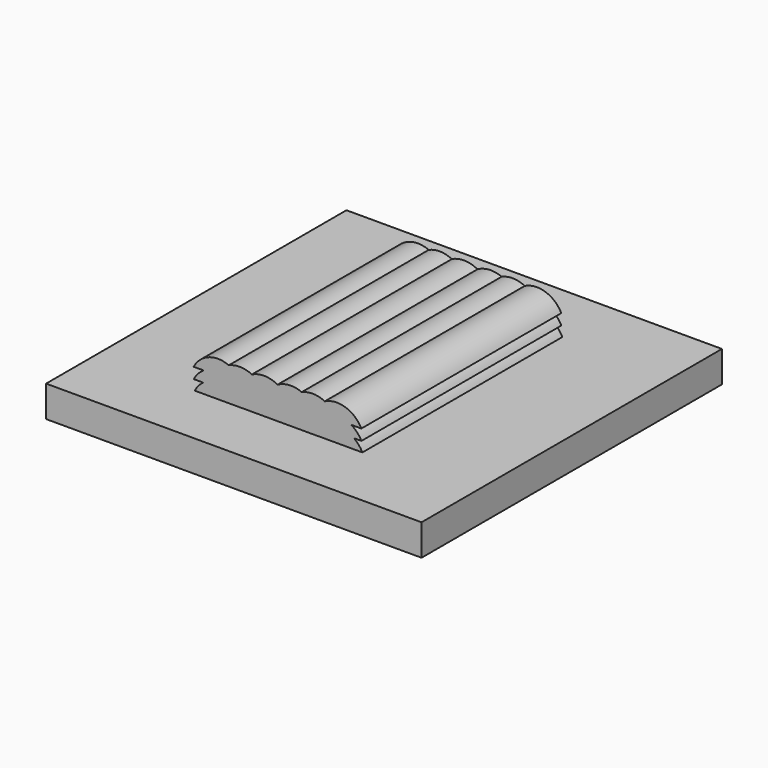
from build123d import *

# Parameters (mm, degrees)
F0_W     = 152.6275277138
F0_H     = 152.6275202632
F1_DEPTH = 12.7
F4_DEPTH = 101.6


with BuildPart() as f1:
    # F0 (on Top) → F1 (new body)
    with BuildSketch(Plane.XY):
        with Locations((0.3492608666, -0.1746304333)):
            Rectangle(F0_W, F0_H)
    extrude(amount=F1_DEPTH)


with BuildPart() as f4:
    # F3 (on offset) → F4 (new body)
    with BuildSketch(Plane.XZ.offset(50.8)):
        with BuildLine():
            ThreePointArc((-23.899851243, 16.6892502457), (-25.8361923758, 14.9089254969), (-27.3004854098, 12.7237895504))
            Line((-27.3004854098, 12.7237895504), (-17.3901738599, 12.7237895504))
            ThreePointArc((-17.3901738599, 12.7237895504), (-15.911695575, 14.925434135), (-13.9541862477, 16.7146502063))
            Line((-13.9541862477, 16.7146502063), (-16.6790850963, 16.7146502063))
            ThreePointArc((-16.6790850963, 16.7146502063), (-16.6725748067, 16.7019543949), (-16.6660808027, 16.6892502457))
            Line((-16.6660808027, 16.6892502457), (-19.7101641502, 16.6892502457))
            Line((-19.7101641502, 16.6892502457), (-23.899851243, 16.6892502457))
        make_face()
        with BuildLine():
            Line((-17.3901738599, 12.7237895504), (-27.3004854098, 12.7237895504))
            ThreePointArc((-27.3004854098, 12.7237895504), (-25.8361923758, 14.9089254969), (-23.899851243, 16.6892502457))
            Line((-23.899851243, 16.6892502457), (-32.6588120256, 16.6892502457))
            ThreePointArc((-32.6588120256, 16.6892502457), (-34.6163213529, 14.9000341745), (-36.0947996378, 12.6983895898))
            Line((-36.0947996378, 12.6983895898), (-16.274176538, 12.6983895898))
            ThreePointArc((-16.274176538, 12.6983895898), (-16.280670542, 12.711093739), (-16.2871808316, 12.7237895504))
            Line((-16.2871808316, 12.7237895504), (-17.3901738599, 12.7237895504))
        make_face()
        with BuildLine():
            ThreePointArc((-13.9541862477, 16.7146502063), (-15.911695575, 14.925434135), (-17.3901738599, 12.7237895504))
            Line((-17.3901738599, 12.7237895504), (-16.2871808316, 12.7237895504))
            Line((-16.2871808316, 12.7237895504), (-7.47986231, 12.7237895504))
            Line((-7.47986231, 12.7237895504), (-6.4638601616, 12.7237895504))
            ThreePointArc((-6.4638601616, 12.7237895504), (-4.9853818767, 14.925434135), (-3.0278725494, 16.7146502063))
            Line((-3.0278725494, 16.7146502063), (-6.8557644263, 16.7146502063))
            Line((-6.8557644263, 16.7146502063), (-7.8717665747, 16.7146502063))
            Line((-7.8717665747, 16.7146502063), (-13.9541862477, 16.7146502063))
        make_face()
        with BuildLine():
            ThreePointArc((-23.8644977976, 16.7146502063), (-23.8821869424, 16.701967516), (-23.899851243, 16.6892502457))
            Line((-23.899851243, 16.6892502457), (-19.7101641502, 16.6892502457))
            ThreePointArc((-19.7101641502, 16.6892502457), (-19.7279755385, 16.7019677558), (-19.7458119078, 16.7146502063))
            Line((-19.7458119078, 16.7146502063), (-23.8644977976, 16.7146502063))
        make_face()
        with BuildLine():
            Line((-32.6588120256, 16.6892502457), (-23.899851243, 16.6892502457))
            ThreePointArc((-23.899851243, 16.6892502457), (-23.8821869424, 16.701967516), (-23.8644977976, 16.7146502063))
            Line((-23.8644977976, 16.7146502063), (-27.6923896745, 16.7146502063))
            ThreePointArc((-27.6923896745, 16.7146502063), (-25.9698422833, 19.1904969058), (-23.6456289265, 21.1127400398))
            Line((-23.6456289265, 21.1127400398), (-32.3987820079, 21.1127400398))
            ThreePointArc((-32.3987820079, 21.1127400398), (-34.7477623291, 19.1828756115), (-36.4867039025, 16.6892502457))
            Line((-36.4867039025, 16.6892502457), (-32.6588120256, 16.6892502457))
        make_face()
        with BuildLine():
            Line((-16.6790850963, 16.7146502063), (-13.9541862477, 16.7146502063))
            Line((-13.9541862477, 16.7146502063), (-7.8717665747, 16.7146502063))
            Line((-7.8717665747, 16.7146502063), (-6.8557644263, 16.7146502063))
            ThreePointArc((-6.8557644263, 16.7146502063), (-5.1168228529, 19.2082755721), (-2.7678425317, 21.1381400004))
            Line((-2.7678425317, 21.1381400004), (-6.8870568648, 21.1381400004))
            Line((-6.8870568648, 21.1381400004), (-7.9030590132, 21.1381400004))
            Line((-7.9030590132, 21.1381400004), (-13.69415623, 21.1381400004))
            ThreePointArc((-13.69415623, 21.1381400004), (-16.0431365512, 19.2082755721), (-17.7820781246, 16.7146502063))
            Line((-17.7820781246, 16.7146502063), (-16.6790850963, 16.7146502063))
        make_face()
        with BuildLine():
            ThreePointArc((-19.7458119078, 16.7146502063), (-19.7279755385, 16.7019677558), (-19.7101641502, 16.6892502457))
            Line((-19.7101641502, 16.6892502457), (-16.6660808027, 16.6892502457))
            ThreePointArc((-16.6660808027, 16.6892502457), (-16.6725748067, 16.7019543949), (-16.6790850963, 16.7146502063))
            Line((-16.6790850963, 16.7146502063), (-17.7820781246, 16.7146502063))
            Line((-17.7820781246, 16.7146502063), (-19.7458119078, 16.7146502063))
        make_face()
        with BuildLine():
            Line((-27.6923896745, 16.7146502063), (-23.8644977976, 16.7146502063))
            Line((-23.8644977976, 16.7146502063), (-19.7458119078, 16.7146502063))
            Line((-19.7458119078, 16.7146502063), (-17.7820781246, 16.7146502063))
            ThreePointArc((-17.7820781246, 16.7146502063), (-16.0431365512, 19.2082755721), (-13.69415623, 21.1381400004))
            Line((-13.69415623, 21.1381400004), (-16.7103775348, 21.1381400004))
            ThreePointArc((-16.7103775348, 21.1381400004), (-16.7038672452, 21.1254441891), (-16.6973732412, 21.1127400398))
            Line((-16.6973732412, 21.1127400398), (-20.7540026972, 21.1127400398))
            Line((-20.7540026972, 21.1127400398), (-23.6456289265, 21.1127400398))
            ThreePointArc((-23.6456289265, 21.1127400398), (-25.9698422833, 19.1904969058), (-27.6923896745, 16.7146502063))
        make_face()
        with BuildLine():
            ThreePointArc((-3.0278725494, 16.7146502063), (-4.9853818767, 14.925434135), (-6.4638601616, 12.7237895504))
            Line((-6.4638601616, 12.7237895504), (2.4304492399, 12.7237895504))
            Line((2.4304492399, 12.7237895504), (13.3567629382, 12.7237895504))
            ThreePointArc((13.3567629382, 12.7237895504), (13.3502689342, 12.7364936996), (13.3437586446, 12.7491895109))
            Line((13.3437586446, 12.7491895109), (12.2407656163, 12.7491895109))
            Line((12.2407656163, 12.7491895109), (2.3304540664, 12.7491895109))
            ThreePointArc((2.3304540664, 12.7491895109), (3.7947471004, 14.9343254574), (5.7310882332, 16.7146502063))
            Line((5.7310882332, 16.7146502063), (2.0385449752, 16.7146502063))
            Line((2.0385449752, 16.7146502063), (-3.0278725494, 16.7146502063))
        make_face()
        with BuildLine():
            ThreePointArc((-2.7678425317, 21.1381400004), (-5.1168228529, 19.2082755721), (-6.8557644263, 16.7146502063))
            Line((-6.8557644263, 16.7146502063), (-3.0278725494, 16.7146502063))
            Line((-3.0278725494, 16.7146502063), (2.0385449752, 16.7146502063))
            ThreePointArc((2.0385449752, 16.7146502063), (2.0320509712, 16.7273543555), (2.0255406816, 16.7400501668))
            Line((2.0255406816, 16.7400501668), (1.9385498017, 16.7400501668))
            ThreePointArc((1.9385498017, 16.7400501668), (1.9601396942, 16.7821320004), (1.9819082764, 16.8241216778))
            ThreePointArc((1.9819082764, 16.8241216778), (3.6931960459, 19.2506339908), (5.9853105497, 21.1381400004))
            Line((5.9853105497, 21.1381400004), (2.0072525367, 21.1381400004))
            Line((2.0072525367, 21.1381400004), (-2.7678425317, 21.1381400004))
        make_face()
        with BuildLine():
            Line((-36.517996341, 21.1127400398), (-32.3987820079, 21.1127400398))
            Line((-32.3987820079, 21.1127400398), (-23.6456289265, 21.1127400398))
            ThreePointArc((-23.6456289265, 21.1127400398), (-23.6250621552, 21.1254623865), (-23.6044677799, 21.1381400004))
            Line((-23.6044677799, 21.1381400004), (-27.723682113, 21.1381400004))
            ThreePointArc((-27.723682113, 21.1381400004), (-25.4303236651, 24.190658722), (-22.2400470078, 26.2881568427))
            ThreePointArc((-22.2400470078, 26.2881568427), (-30.3993259782, 26.515265819), (-36.517996341, 21.1127400398))
        make_face()
        with BuildLine():
            ThreePointArc((-23.6044677799, 21.1381400004), (-23.6250621552, 21.1254623865), (-23.6456289265, 21.1127400398))
            Line((-23.6456289265, 21.1127400398), (-20.7540026972, 21.1127400398))
            ThreePointArc((-20.7540026972, 21.1127400398), (-20.7747717042, 21.1254627675), (-20.7955685121, 21.1381400004))
            Line((-20.7955685121, 21.1381400004), (-23.6044677799, 21.1381400004))
        make_face()
        with BuildLine():
            Line((-16.7103775348, 21.1381400004), (-13.69415623, 21.1381400004))
            Line((-13.69415623, 21.1381400004), (-7.9030590132, 21.1381400004))
            Line((-7.9030590132, 21.1381400004), (-6.8870568648, 21.1381400004))
            ThreePointArc((-6.8870568648, 21.1381400004), (-5.0052271885, 23.7835064069), (-2.439902164, 25.7730676333))
            ThreePointArc((-2.439902164, 25.7730676333), (-7.6155816808, 27.2029401673), (-12.8582147881, 26.0423403114))
            ThreePointArc((-12.8582147881, 26.0423403114), (-15.7298287727, 23.9883703542), (-17.8133705631, 21.1381400004))
            Line((-17.8133705631, 21.1381400004), (-16.7103775348, 21.1381400004))
        make_face()
        with BuildLine():
            Line((-6.8870568648, 21.1381400004), (-2.7678425317, 21.1381400004))
            Line((-2.7678425317, 21.1381400004), (2.0072525367, 21.1381400004))
            ThreePointArc((2.0072525367, 21.1381400004), (2.0007585327, 21.1508441496), (1.9942482431, 21.163539961))
            Line((1.9942482431, 21.163539961), (1.9072573632, 21.163539961))
            ThreePointArc((1.9072573632, 21.163539961), (1.9288472557, 21.2056217946), (1.9506158379, 21.247611472))
            ThreePointArc((1.9506158379, 21.247611472), (4.2351608696, 24.2483641482), (7.3908924684, 26.3135568032))
            ThreePointArc((7.3908924684, 26.3135568032), (2.4124579582, 27.1898767431), (-2.439902164, 25.7730676333))
            ThreePointArc((-2.439902164, 25.7730676333), (-5.0052271885, 23.7835064069), (-6.8870568648, 21.1381400004))
        make_face()
        with BuildLine():
            ThreePointArc((-20.7955685121, 21.1381400004), (-20.7747717042, 21.1254627675), (-20.7540026972, 21.1127400398))
            Line((-20.7540026972, 21.1127400398), (-16.6973732412, 21.1127400398))
            ThreePointArc((-16.6973732412, 21.1127400398), (-16.7038672452, 21.1254441891), (-16.7103775348, 21.1381400004))
            Line((-16.7103775348, 21.1381400004), (-17.8133705631, 21.1381400004))
            Line((-17.8133705631, 21.1381400004), (-20.7955685121, 21.1381400004))
        make_face()
        with BuildLine():
            Line((-27.723682113, 21.1381400004), (-23.6044677799, 21.1381400004))
            Line((-23.6044677799, 21.1381400004), (-20.7955685121, 21.1381400004))
            Line((-20.7955685121, 21.1381400004), (-17.8133705631, 21.1381400004))
            ThreePointArc((-17.8133705631, 21.1381400004), (-15.7298287727, 23.9883703542), (-12.8582147881, 26.0423403114))
            ThreePointArc((-12.8582147881, 26.0423403114), (-17.5219446851, 27.2028374115), (-22.2400470078, 26.2881568427))
            ThreePointArc((-22.2400470078, 26.2881568427), (-25.4303236651, 24.190658722), (-27.723682113, 21.1381400004))
        make_face()
        with BuildLine():
            ThreePointArc((2.0255406816, 16.7400501668), (2.0320509712, 16.7273543555), (2.0385449752, 16.7146502063))
            Line((2.0385449752, 16.7146502063), (5.7310882332, 16.7146502063))
            ThreePointArc((5.7310882332, 16.7146502063), (5.7487525338, 16.7273674766), (5.7664416786, 16.7400501668))
            Line((5.7664416786, 16.7400501668), (2.0255406816, 16.7400501668))
        make_face()
        with BuildLine():
            ThreePointArc((1.9942482431, 21.163539961), (2.0007585327, 21.1508441496), (2.0072525367, 21.1381400004))
            Line((2.0072525367, 21.1381400004), (5.9853105497, 21.1381400004))
            ThreePointArc((5.9853105497, 21.1381400004), (6.005877321, 21.1508623471), (6.0264716963, 21.163539961))
            Line((6.0264716963, 21.163539961), (1.9942482431, 21.163539961))
        make_face()
        with BuildLine():
            Line((12.2407656163, 12.7491895109), (13.3437586446, 12.7491895109))
            Line((13.3437586446, 12.7491895109), (22.1510771662, 12.7491895109))
            Line((22.1510771662, 12.7491895109), (32.0613887161, 12.7491895109))
            ThreePointArc((32.0613887161, 12.7491895109), (30.5829104312, 14.9508340956), (28.6254011039, 16.7400501668))
            Line((28.6254011039, 16.7400501668), (21.7591729015, 16.7400501668))
            Line((21.7591729015, 16.7400501668), (15.6767532285, 16.7400501668))
            ThreePointArc((15.6767532285, 16.7400501668), (13.7192439012, 14.9508340956), (12.2407656163, 12.7491895109))
        make_face()
        with BuildLine():
            Line((1.9385498017, 16.7400501668), (2.0255406816, 16.7400501668))
            ThreePointArc((2.0255406816, 16.7400501668), (2.0038139428, 16.7821323533), (1.9819082764, 16.8241216778))
            ThreePointArc((1.9819082764, 16.8241216778), (1.9601396942, 16.7821320004), (1.9385498017, 16.7400501668))
        make_face()
        with BuildLine():
            ThreePointArc((1.9819082764, 16.8241216778), (2.0038139428, 16.7821323533), (2.0255406816, 16.7400501668))
            Line((2.0255406816, 16.7400501668), (5.7664416786, 16.7400501668))
            Line((5.7664416786, 16.7400501668), (9.8851275684, 16.7400501668))
            Line((9.8851275684, 16.7400501668), (11.8488613516, 16.7400501668))
            ThreePointArc((11.8488613516, 16.7400501668), (13.587802925, 19.2336755327), (15.9367832462, 21.163539961))
            Line((15.9367832462, 21.163539961), (12.9205619414, 21.163539961))
            ThreePointArc((12.9205619414, 21.163539961), (12.927072231, 21.1508441496), (12.933566235, 21.1381400004))
            Line((12.933566235, 21.1381400004), (8.876936779, 21.1381400004))
            Line((8.876936779, 21.1381400004), (5.9853105497, 21.1381400004))
            ThreePointArc((5.9853105497, 21.1381400004), (3.6931960459, 19.2506339908), (1.9819082764, 16.8241216778))
        make_face()
        with BuildLine():
            ThreePointArc((5.7664416786, 16.7400501668), (5.7487525338, 16.7273674766), (5.7310882332, 16.7146502063))
            Line((5.7310882332, 16.7146502063), (9.920775326, 16.7146502063))
            ThreePointArc((9.920775326, 16.7146502063), (9.9029639377, 16.7273677164), (9.8851275684, 16.7400501668))
            Line((9.8851275684, 16.7400501668), (5.7664416786, 16.7400501668))
        make_face()
        with BuildLine():
            Line((9.920775326, 16.7146502063), (5.7310882332, 16.7146502063))
            ThreePointArc((5.7310882332, 16.7146502063), (3.7947471004, 14.9343254574), (2.3304540664, 12.7491895109))
            Line((2.3304540664, 12.7491895109), (12.2407656163, 12.7491895109))
            ThreePointArc((12.2407656163, 12.7491895109), (13.7192439012, 14.9508340956), (15.6767532285, 16.7400501668))
            Line((15.6767532285, 16.7400501668), (12.9518543799, 16.7400501668))
            ThreePointArc((12.9518543799, 16.7400501668), (12.9583646695, 16.7273543555), (12.9648586735, 16.7146502063))
            Line((12.9648586735, 16.7146502063), (9.920775326, 16.7146502063))
        make_face()
        with BuildLine():
            Line((1.9072573632, 21.163539961), (1.9942482431, 21.163539961))
            ThreePointArc((1.9942482431, 21.163539961), (1.9725215042, 21.2056221474), (1.9506158379, 21.247611472))
            ThreePointArc((1.9506158379, 21.247611472), (1.9288472557, 21.2056217946), (1.9072573632, 21.163539961))
        make_face()
        with BuildLine():
            ThreePointArc((1.9506158379, 21.247611472), (1.9725215042, 21.2056221474), (1.9942482431, 21.163539961))
            Line((1.9942482431, 21.163539961), (6.0264716963, 21.163539961))
            Line((6.0264716963, 21.163539961), (8.8353709641, 21.163539961))
            Line((8.8353709641, 21.163539961), (11.8175689131, 21.163539961))
            ThreePointArc((11.8175689131, 21.163539961), (13.9011107034, 24.0137703148), (16.7727246881, 26.067740272))
            ThreePointArc((16.7727246881, 26.067740272), (12.1089947911, 27.2282373721), (7.3908924684, 26.3135568032))
            ThreePointArc((7.3908924684, 26.3135568032), (4.2351608696, 24.2483641482), (1.9506158379, 21.247611472))
        make_face()
        with BuildLine():
            ThreePointArc((6.0264716963, 21.163539961), (6.005877321, 21.1508623471), (5.9853105497, 21.1381400004))
            Line((5.9853105497, 21.1381400004), (8.876936779, 21.1381400004))
            ThreePointArc((8.876936779, 21.1381400004), (8.856167772, 21.150862728), (8.8353709641, 21.163539961))
            Line((8.8353709641, 21.163539961), (6.0264716963, 21.163539961))
        make_face()
        with BuildLine():
            ThreePointArc((9.8851275684, 16.7400501668), (9.9029639377, 16.7273677164), (9.920775326, 16.7146502063))
            Line((9.920775326, 16.7146502063), (12.9648586735, 16.7146502063))
            ThreePointArc((12.9648586735, 16.7146502063), (12.9583646695, 16.7273543555), (12.9518543799, 16.7400501668))
            Line((12.9518543799, 16.7400501668), (11.8488613516, 16.7400501668))
            Line((11.8488613516, 16.7400501668), (9.8851275684, 16.7400501668))
        make_face()
        with BuildLine():
            ThreePointArc((8.8353709641, 21.163539961), (8.856167772, 21.150862728), (8.876936779, 21.1381400004))
            Line((8.876936779, 21.1381400004), (12.933566235, 21.1381400004))
            ThreePointArc((12.933566235, 21.1381400004), (12.927072231, 21.1508441496), (12.9205619414, 21.163539961))
            Line((12.9205619414, 21.163539961), (11.8175689131, 21.163539961))
            Line((11.8175689131, 21.163539961), (8.8353709641, 21.163539961))
        make_face()
        with BuildLine():
            Line((12.9518543799, 16.7400501668), (15.6767532285, 16.7400501668))
            Line((15.6767532285, 16.7400501668), (21.7591729015, 16.7400501668))
            Line((21.7591729015, 16.7400501668), (28.6254011039, 16.7400501668))
            Line((28.6254011039, 16.7400501668), (31.6694844514, 16.7400501668))
            ThreePointArc((31.6694844514, 16.7400501668), (29.930542878, 19.2336755327), (27.5815625569, 21.163539961))
            Line((27.5815625569, 21.163539961), (21.727880463, 21.163539961))
            Line((21.727880463, 21.163539961), (15.9367832462, 21.163539961))
            ThreePointArc((15.9367832462, 21.163539961), (13.587802925, 19.2336755327), (11.8488613516, 16.7400501668))
            Line((11.8488613516, 16.7400501668), (12.9518543799, 16.7400501668))
        make_face()
        with BuildLine():
            ThreePointArc((31.6381920129, 21.163539961), (25.2137357901, 26.6719009504), (16.7727246881, 26.067740272))
            ThreePointArc((16.7727246881, 26.067740272), (13.9011107034, 24.0137703148), (11.8175689131, 21.163539961))
            Line((11.8175689131, 21.163539961), (12.9205619414, 21.163539961))
            Line((12.9205619414, 21.163539961), (15.9367832462, 21.163539961))
            Line((15.9367832462, 21.163539961), (21.727880463, 21.163539961))
            Line((21.727880463, 21.163539961), (27.5815625569, 21.163539961))
            Line((27.5815625569, 21.163539961), (31.6381920129, 21.163539961))
        make_face()
    extrude(amount=-F4_DEPTH)


solid = Compound([f1.part, f4.part])
